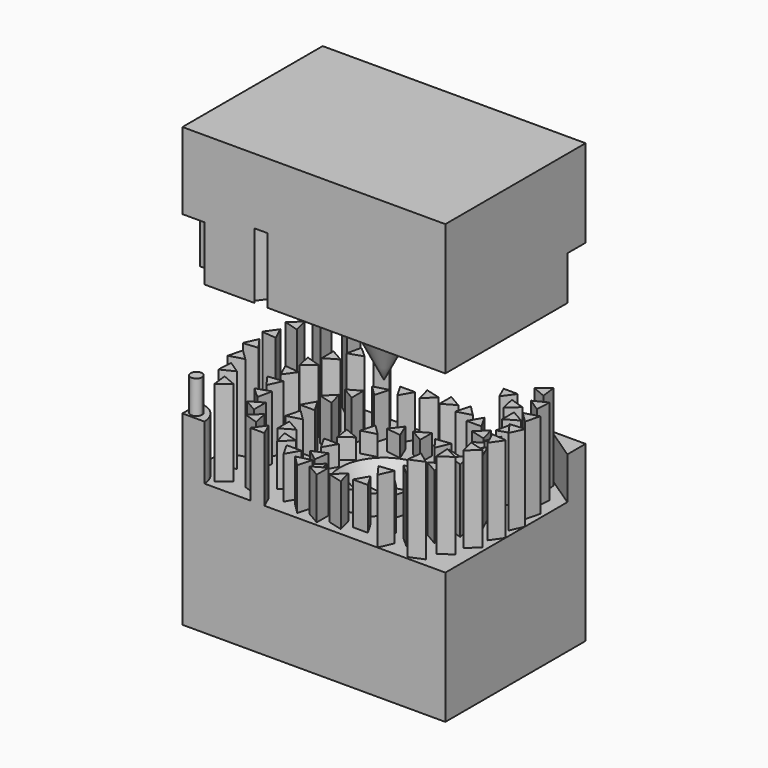
from build123d import *

# Parameters (mm, degrees)
F0_W      = 76.2
F0_H      = 50.8
F1_DEPTH  = 38.1
F3_W      = 76.2
F3_H      = 50.8
F4_DEPTH  = 38.1
F5_R      = 12.192
F13_DEPTH = 6.35
F16_DEPTH = 12.7
F17_DEPTH = 19.05
F18_DEPTH = 25.4
F20_DEPTH = 15.875
F21_DEPTH = 25.908
F23_DEPTH = 25.4
F24_DEPTH = 15.8242
F26_DEPTH = 12.7
F29_DEPTH = 5.842
F30_DEPTH = 12.192
F31_DEPTH = 18.542
F32_DEPTH = 24.892
F33_DEPTH = 12.192


# Not quite as in the source:
# - a feature names something its author has since deleted; it is built from what else it names


with BuildPart() as f1:
    # F0 (on Top) → F1 (new body)
    with BuildSketch(Plane.XY):
        Rectangle(F0_W, F0_H)
    extrude(amount=F1_DEPTH)

    # F14 (on 3pt) → F15 (revolve, cut)
    with BuildSketch(Plane(origin=(0, 0, 0), x_dir=(0, -1, 0), z_dir=(-1, 0, 0))):
        Polygon((0, 12.7), (0, 38.0711555481), (0, 38.1), (-12.7, 38.1), align=None)
    revolve(axis=Axis((0, 0, 25.4), (0, 0, -1)), mode=Mode.SUBTRACT)

    # F22 (on face) → F23 (join)
    with BuildSketch(Plane.XY.offset(38.1)):
        with BuildLine():
            Line((-37.0223692655, -24.3223692655), (-34.687502674, -21.987502674))
            ThreePointArc((-34.687502674, -21.987502674), (-37.0223692655, -21.987502674), (-37.0223692655, -24.3223692655))
        make_face()
        with BuildLine():
            ThreePointArc((-34.2039359697, -23.1549359697), (-34.3296108616, -22.5231256229), (-34.687502674, -21.987502674))
            Line((-34.687502674, -21.987502674), (-37.0223692655, -24.3223692655))
            ThreePointArc((-37.0223692655, -24.3223692655), (-35.2231256229, -24.6802610779), (-34.2039359697, -23.1549359697))
        make_face()
    extrude(amount=F23_DEPTH)

    # F22 (on face) → F24 (join)
    with BuildSketch(Plane.XY.offset(38.1)):
        with BuildLine():
            Line((-34.687502674, -21.987502674), (-33.6098719395, -20.9098719395))
            ThreePointArc((-33.6098719395, -20.9098719395), (-35.6699602045, -19.5333649686), (-38.1, -19.05))
            Line((-38.1, -19.05), (-38.1, -25.4))
            Line((-38.1, -25.4), (-37.0223692655, -24.3223692655))
            ThreePointArc((-37.0223692655, -24.3223692655), (-37.0223692655, -21.987502674), (-34.687502674, -21.987502674))
        make_face()
        with BuildLine():
            Line((-38.1, -25.4), (-31.75, -25.4))
            ThreePointArc((-31.75, -25.4), (-32.2333649686, -22.9699602045), (-33.6098719395, -20.9098719395))
            Line((-33.6098719395, -20.9098719395), (-34.687502674, -21.987502674))
            ThreePointArc((-34.687502674, -21.987502674), (-34.3296108616, -22.5231256229), (-34.2039359697, -23.1549359697))
            ThreePointArc((-34.2039359697, -23.1549359697), (-35.2231256229, -24.6802610779), (-37.0223692655, -24.3223692655))
            Line((-37.0223692655, -24.3223692655), (-38.1, -25.4))
        make_face()
    extrude(amount=F24_DEPTH)

    # F28 (on face) → F29 (join)
    with BuildSketch(Plane.XY.offset(38.1)):
        Polygon((-5.0058819788, 12.0852681648), (-6.6583090397, 16.0745799862), (-9.2869408902, 12.6488802628), align=None)
        Polygon((-9.2496638047, 9.2496638047), (-12.3029508859, 12.3029508859), (-13.4205315226, 8.1320831679), align=None)
        Polygon((5.0058819788, 12.0852681648), (6.6583090397, 16.0745799862), (2.3772501283, 15.5109678882), align=None)
        Polygon((9.2496638047, 9.2496638047), (12.3029508859, 12.3029508859), (8.1320831679, 13.4205315226), align=None)
        Polygon((12.0852681648, -5.0058819788), (16.0745799862, -6.6583090397), (15.5109678882, -2.3772501283), align=None)
        Polygon((12.0852681648, 5.0058819788), (16.0745799862, 6.6583090397), (12.6488802628, 9.2869408902), align=None)
        Polygon((13.081, 0), (17.399, 0), (15.24, 3.7394976935), align=None)
        Polygon((9.2496638047, -9.2496638047), (12.3029508859, -12.3029508859), (13.4205315226, -8.1320831679), align=None)
        Polygon((5.0058819788, -12.0852681648), (6.6583090397, -16.0745799862), (9.2869408902, -12.6488802628), align=None)
        Polygon((0, -13.081), (0, -17.399), (3.7394976935, -15.24), align=None)
        Polygon((-5.0058819788, -12.0852681648), (-6.6583090397, -16.0745799862), (-2.3772501283, -15.5109678882), align=None)
        Polygon((-9.2496638047, -9.2496638047), (-12.3029508859, -12.3029508859), (-8.1320831679, -13.4205315226), align=None)
        Polygon((-12.0852681648, -5.0058819788), (-16.0745799862, -6.6583090397), (-12.6488802628, -9.2869408902), align=None)
        Polygon((-13.081, 0), (-17.399, 0), (-15.24, -3.7394976935), align=None)
        Polygon((-12.0852681648, 5.0058819788), (-16.0745799862, 6.6583090397), (-15.5109678882, 2.3772501283), align=None)
        Polygon((-3.7394976935, 15.24), (0, 13.081), (0, 17.399), align=None)
    extrude(amount=F29_DEPTH)

    # F28 (on face) → F30 (join)
    with BuildSketch(Plane.XY.offset(38.1)):
        Polygon((-19.3822676303, 5.193462959), (-20.4998482671, 9.3643306769), (-23.5531353482, 6.3110435958), align=None)
        Polygon((-17.3776657523, 10.033), (-17.3776657523, 14.351), (-21.1171634459, 12.192), align=None)
        Polygon((-14.1888046713, 14.1888046713), (-13.0712240345, 18.3596723892), (-17.2420917525, 17.2420917525), align=None)
        Polygon((-20.066, 0), (-22.225, 3.7394976935), (-24.384, 0), align=None)
        Polygon((-19.3822676303, -5.193462959), (-22.4355547115, -2.1401758779), (-23.5531353482, -6.3110435958), align=None)
        Polygon((-17.3776657523, -10.033), (-21.1171634459, -7.874), (-21.1171634459, -12.192), align=None)
        Polygon((-14.1888046713, -14.1888046713), (-18.3596723892, -13.0712240345), (-17.2420917525, -17.2420917525), align=None)
        Polygon((-10.033, -17.3776657523), (-14.351, -17.3776657523), (-12.192, -21.1171634459), align=None)
        Polygon((-5.193462959, -19.3822676303), (-9.3643306769, -20.4998482671), (-6.3110435958, -23.5531353482), align=None)
        Polygon((-10.033, 17.3776657523), (-7.874, 21.1171634459), (-12.192, 21.1171634459), align=None)
        Polygon((-5.193462959, 19.3822676303), (-2.1401758779, 22.4355547115), (-6.3110435958, 23.5531353482), align=None)
        Polygon((0, 24.384), (0, 20.066), (3.7394976935, 22.225), align=None)
        Polygon((5.193462959, 19.3822676303), (9.3643306769, 20.4998482671), (6.3110435958, 23.5531353482), align=None)
        Polygon((10.033, 17.3776657523), (14.351, 17.3776657523), (12.192, 21.1171634459), align=None)
        Polygon((14.1888046713, 14.1888046713), (18.3596723892, 13.0712240345), (17.2420917525, 17.2420917525), align=None)
        Polygon((17.3776657523, 10.033), (21.1171634459, 7.874), (21.1171634459, 12.192), align=None)
        Polygon((19.3822676303, 5.193462959), (22.4355547115, 2.1401758779), (23.5531353482, 6.3110435958), align=None)
        Polygon((20.066, 0), (22.225, -3.7394976935), (24.384, 0), align=None)
        Polygon((19.3822676303, -5.193462959), (20.4998482671, -9.3643306769), (23.5531353482, -6.3110435958), align=None)
        Polygon((17.3776657523, -10.033), (17.3776657523, -14.351), (21.1171634459, -12.192), align=None)
        Polygon((14.1888046713, -14.1888046713), (13.0712240345, -18.3596723892), (17.2420917525, -17.2420917525), align=None)
        Polygon((10.033, -17.3776657523), (7.874, -21.1171634459), (12.192, -21.1171634459), align=None)
        Polygon((5.193462959, -19.3822676303), (2.1401758779, -22.4355547115), (6.3110435958, -23.5531353482), align=None)
        Polygon((0, -20.066), (-3.7394976935, -22.225), (0, -24.384), align=None)
    extrude(amount=F30_DEPTH)

    # F28 (on face) → F31 (join)
    with BuildSketch(Plane.XY.offset(38.1)):
        Polygon((18.2294342554, 25.4), (14.3350747947, 25.4), (15.9001788598, 21.8847187148), (18.4382355792, 25.3780540965), align=None)
        Polygon((19.205047993, 22.3242933726), (20.102810674, 18.1006520326), (23.3117100304, 20.9899579909), align=None)
        Polygon((23.4268531978, 17.8435), (23.4268531978, 13.5255), (27.1663508913, 15.6845), align=None)
        Polygon((26.6247925033, 12.5828600548), (25.7270298223, 8.3592187148), (29.8336918597, 9.6935540965), align=None)
        Polygon((28.6591006164, 6.772288746), (26.9028117916, 2.8275994599), (31.1971573358, 3.2789533642), align=None)
        Polygon((29.440868511, 0.6657359219), (26.9028117916, -2.8275994599), (31.1971573358, -3.2789533642), align=None)
        Polygon((28.9359291787, -5.4699127566), (25.7270298223, -8.3592187148), (29.8336918597, -9.6935540965), align=None)
        Polygon((27.1663508913, -11.3665), (23.4268531978, -13.5255), (27.1663508913, -15.6845), align=None)
        Polygon((24.2094727114, -16.7663166509), (20.102810674, -18.1006520326), (23.3117100304, -20.9899579909), align=None)
        Polygon((20.194524404, -21.4333648104), (15.9001788598, -21.8847187148), (18.4382355792, -25.3780540965), align=None)
        Polygon((-18.4382355792, -25.3780540965), (-18.2294342554, -25.4), (-14.3350747947, -25.4), (-15.9001788598, -21.8847187148), align=None)
        Polygon((-19.205047993, -22.3242933726), (-20.102810674, -18.1006520326), (-23.3117100304, -20.9899579909), align=None)
        Polygon((-23.4268531978, -17.8435), (-23.4268531978, -13.5255), (-27.1663508913, -15.6845), align=None)
        Polygon((-26.6247925033, -12.5828600548), (-25.7270298223, -8.3592187148), (-29.8336918597, -9.6935540965), align=None)
        Polygon((-28.6591006164, -6.772288746), (-26.9028117916, -2.8275994599), (-31.1971573358, -3.2789533642), align=None)
        Polygon((-29.440868511, -0.6657359219), (-26.9028117916, 2.8275994599), (-31.1971573358, 3.2789533642), align=None)
        Polygon((-28.9359291787, 5.4699127566), (-25.7270298223, 8.3592187148), (-29.8336918597, 9.6935540965), align=None)
        Polygon((-27.1663508913, 11.3665), (-23.4268531978, 13.5255), (-27.1663508913, 15.6845), align=None)
        Polygon((-24.2094727114, 16.7663166509), (-20.102810674, 18.1006520326), (-23.3117100304, 20.9899579909), align=None)
        Polygon((-20.194524404, 21.4333648104), (-15.9001788598, 21.8847187148), (-18.4382355792, 25.3780540965), align=None)
    extrude(amount=F31_DEPTH)

    # F28 (on face) → F32 (join)
    with BuildSketch(Plane.XY.offset(38.1)):
        Polygon((-27.1613143477, 20.5112724838), (-26.6306827086, 24.7965442446), (-30.6071527351, 23.1134488437), align=None)
        Polygon((-30.4677777846, 15.1711506772), (-30.7335977772, 19.4809608507), (-34.3330928766, 17.0958488975), align=None)
        Polygon((-32.736697591, 9.3143935301), (-33.7899170345, 13.5019766999), (-36.8898607183, 10.4960703212), align=None)
        Polygon((-35.6955611936, 7.0631989264), (-38.1, 3.666548848), (-38.1, 3.5304849218), (-33.8908084244, 3.1404458827), align=None)
        Polygon((-36.3856358284, 0.3838923849), (-38.1, -3.3423948867), (-38.1, -3.5304849218), (-33.8908084244, -3.1404458827), align=None)
        Polygon((-32.736697591, -9.3143935301), (-35.8366412748, -6.3084871514), (-36.8898607183, -10.4960703212), align=None)
        Polygon((-30.4677777846, -15.1711506772), (-34.0672728839, -12.786038724), (-34.3330928766, -17.0958488975), align=None)
        Polygon((-27.1613143477, -20.5112724838), (-31.1377843742, -18.8281770829), (-30.6071527351, -23.1134488437), align=None)
        Polygon((27.1613143477, -20.5112724838), (26.6306827086, -24.7965442446), (30.6071527351, -23.1134488437), align=None)
        Polygon((30.4677777846, -15.1711506772), (30.7335977772, -19.4809608507), (34.3330928766, -17.0958488975), align=None)
        Polygon((32.736697591, -9.3143935301), (33.7899170345, -13.5019766999), (36.8898607183, -10.4960703212), align=None)
        Polygon((38.1, -3.666548848), (38.1, -3.5304849218), (33.8908084244, -3.1404458827), (35.6955611936, -7.0631989264), align=None)
        Polygon((38.1, 3.3423948867), (38.1, 3.5304849218), (33.8908084244, 3.1404458827), (36.3856358284, -0.3838923849), align=None)
        Polygon((32.736697591, 9.3143935301), (35.8366412748, 6.3084871514), (36.8898607183, 10.4960703212), align=None)
        Polygon((30.4677777846, 15.1711506772), (34.0672728839, 12.786038724), (34.3330928766, 17.0958488975), align=None)
        Polygon((27.1613143477, 20.5112724838), (31.1377843742, 18.8281770829), (30.6071527351, 23.1134488437), align=None)
    extrude(amount=F32_DEPTH)

    # F27 (on face) → F33 (join)
    with BuildSketch(Plane.XY.offset(38.1)):
        Polygon((38.1, 25.4), (28.2770834, 25.4), (38.1, 18.796), align=None)
    extrude(amount=F33_DEPTH)


with BuildPart() as f4:
    # F3 (on offset) → F4 (new body)
    with BuildSketch(Plane.XY.offset(127)):
        Rectangle(F3_W, F3_H)
    extrude(amount=-F4_DEPTH)

    # F5 (on face) → F8 section 0
    with BuildSketch(Plane(origin=(0, 0, 88.9), x_dir=(1, 0, 0), z_dir=(0, 0, -1)), mode=Mode.PRIVATE) as f8_s0:
        Circle(F5_R)
    loft([f8_s0.sketch, Vertex(0, 0, 64.516)])

    # F12 (on face) → F13 (cut)
    with BuildSketch(Plane(origin=(0, 0, 88.9), x_dir=(1, 0, 0), z_dir=(0, 0, -1))):
        Polygon((0, 17.272), (0, 12.192), (4.3994090512, 14.732), align=None)
        Polygon((-6.6097082438, 15.9572472855), (-4.6656764074, 11.2639392604), (-1.573168348, 15.2941742291), align=None)
        Polygon((-12.2131483247, 12.2131483247), (-8.6210458762, 8.6210458762), (-7.3062451271, 13.5279490738), align=None)
        Polygon((-15.9572472855, 6.6097082438), (-11.2639392604, 4.6656764074), (-11.9270123169, 9.7022163032), align=None)
        Polygon((-17.272, 0), (-12.192, 0), (-14.732, 4.3994090512), align=None)
        Polygon((-15.9572472855, -6.6097082438), (-11.2639392604, -4.6656764074), (-15.2941742291, -1.573168348), align=None)
        Polygon((-12.2131483247, -12.2131483247), (-8.6210458762, -8.6210458762), (-13.5279490738, -7.3062451271), align=None)
        Polygon((-6.6097082438, -15.9572472855), (-4.6656764074, -11.2639392604), (-9.7022163032, -11.9270123169), align=None)
        Polygon((0, -17.272), (0, -12.192), (-4.3994090512, -14.732), align=None)
        Polygon((6.6097082438, -15.9572472855), (4.6656764074, -11.2639392604), (1.573168348, -15.2941742291), align=None)
        Polygon((12.2131483247, -12.2131483247), (8.6210458762, -8.6210458762), (7.3062451271, -13.5279490738), align=None)
        Polygon((15.9572472855, -6.6097082438), (11.2639392604, -4.6656764074), (11.9270123169, -9.7022163032), align=None)
        Polygon((15.9572472855, 6.6097082438), (11.2639392604, 4.6656764074), (15.2941742291, 1.573168348), align=None)
        Polygon((17.272, 0), (12.192, 0), (14.732, -4.3994090512), align=None)
        Polygon((12.2131483247, 12.2131483247), (8.6210458762, 8.6210458762), (13.5279490738, 7.3062451271), align=None)
        Polygon((6.6097082438, 15.9572472855), (4.6656764074, 11.2639392604), (9.7022163032, 11.9270123169), align=None)
    extrude(amount=-F13_DEPTH, mode=Mode.SUBTRACT)

    # F12 (on face) → F16 (cut)
    with BuildSketch(Plane(origin=(0, 0, 88.9), x_dir=(1, 0, 0), z_dir=(0, 0, -1))):
        Polygon((-4.9633728279, 18.5235595707), (-6.2781735771, 23.4304627683), (-9.8702760255, 19.8383603199), align=None)
        Polygon((-9.5885, 16.6077691684), (-12.1285, 21.0071782196), (-14.6685, 16.6077691684), align=None)
        Polygon((-13.5601867428, 13.5601867428), (-17.1522891912, 17.1522891912), (-18.4670899404, 12.2453859937), align=None)
        Polygon((-16.6077691684, 9.5885), (-21.0071782196, 12.1285), (-21.0071782196, 7.0485), align=None)
        Polygon((-18.5235595707, 4.9633728279), (-23.4304627683, 6.2781735771), (-22.1156620192, 1.3712703795), align=None)
        Polygon((-19.177, 0), (-24.257, 0), (-21.717, -4.3994090512), align=None)
        Polygon((-18.5235595707, -4.9633728279), (-23.4304627683, -6.2781735771), (-19.8383603199, -9.8702760255), align=None)
        Polygon((-16.6077691684, -9.5885), (-21.0071782196, -12.1285), (-16.6077691684, -14.6685), align=None)
        Polygon((-13.5601867428, -13.5601867428), (-17.1522891912, -17.1522891912), (-12.2453859937, -18.4670899404), align=None)
        Polygon((-9.5885, -16.6077691684), (-12.1285, -21.0071782196), (-7.0485, -21.0071782196), align=None)
        Polygon((-4.9633728279, -18.5235595707), (-6.2781735771, -23.4304627683), (-1.3712703795, -22.1156620192), align=None)
        Polygon((0, -19.177), (0, -24.257), (4.3994090512, -21.717), align=None)
        Polygon((4.9633728279, -18.5235595707), (6.2781735771, -23.4304627683), (9.8702760255, -19.8383603199), align=None)
        Polygon((9.5885, -16.6077691684), (12.1285, -21.0071782196), (14.6685, -16.6077691684), align=None)
        Polygon((13.5601867428, -13.5601867428), (17.1522891912, -17.1522891912), (18.4670899404, -12.2453859937), align=None)
        Polygon((16.6077691684, -9.5885), (21.0071782196, -12.1285), (21.0071782196, -7.0485), align=None)
        Polygon((4.9633728279, 18.5235595707), (6.2781735771, 23.4304627683), (1.3712703795, 22.1156620192), align=None)
        Polygon((9.5885, 16.6077691684), (12.1285, 21.0071782196), (7.0485, 21.0071782196), align=None)
        Polygon((13.5601867428, 13.5601867428), (17.1522891912, 17.1522891912), (12.2453859937, 18.4670899404), align=None)
        Polygon((16.6077691684, 9.5885), (21.0071782196, 12.1285), (16.6077691684, 14.6685), align=None)
        Polygon((18.5235595707, 4.9633728279), (23.4304627683, 6.2781735771), (19.8383603199, 9.8702760255), align=None)
        Polygon((19.177, 0), (24.257, 0), (21.717, 4.3994090512), align=None)
        Polygon((18.5235595707, -4.9633728279), (23.4304627683, -6.2781735771), (22.1156620192, -1.3712703795), align=None)
        Polygon((-4.3994090512, 21.717), (0, 19.177), (0, 24.257), align=None)
    extrude(amount=-F16_DEPTH, mode=Mode.SUBTRACT)

    # F12 (on face) → F17 (cut)
    with BuildSketch(Plane(origin=(0, 0, 88.9), x_dir=(1, 0, 0), z_dir=(0, 0, -1))):
        Polygon((-15.3776377705, 21.1655026068), (-13.4923180632, 25.4), (-17.1772306466, 25.4), (-18.3635868521, 25.2753089383), align=None)
        Polygon((12.707266203, 28.5409871877), (11.3088086068, 25.4), (14.9893269747, 25.4), align=None)
        Polygon((13.4923180632, -25.4), (17.1772306466, -25.4), (18.3635868521, -25.2753089383), (15.3776377705, -21.1655026068), align=None)
        Polygon((-23.2173306376, 20.9049784039), (-19.4421549241, 17.5057949236), (-18.3859635348, 22.4747847353), align=None)
        Polygon((-27.056365665, 15.621), (-22.6569566138, 13.081), (-22.6569566138, 18.161), align=None)
        Polygon((-29.7129076821, 9.6543089383), (-24.8815405793, 8.0845026068), (-25.9377319687, 13.0534924186), align=None)
        Polygon((-31.0708530551, 3.2656782494), (-26.0186818266, 2.734673656), (-28.0849039734, 7.3754845808), align=None)
        Polygon((-31.0708530551, -3.2656782494), (-26.0186818266, -2.734673656), (-29.0046309083, 1.3751326754), align=None)
        Polygon((-29.7129076821, -9.6543089383), (-24.8815405793, -8.0845026068), (-28.6567162927, -4.6853191265), align=None)
        Polygon((-27.056365665, -15.621), (-22.6569566138, -13.081), (-27.056365665, -10.541), align=None)
        Polygon((-23.2173306376, -20.9049784039), (-19.4421549241, -17.5057949236), (-24.2735220269, -15.9359885921), align=None)
        Polygon((-18.3635868521, -25.2753089383), (-15.3776377705, -21.1655026068), (-20.4298089989, -20.6344980134), align=None)
        Polygon((-6.4955770445, -30.5592873421), (-5.4393856552, -25.5902975304), (-10.270752758, -27.1601038618), align=None)
        Polygon((23.2173306376, -20.9049784039), (19.4421549241, -17.5057949236), (18.3859635348, -22.4747847353), align=None)
        Polygon((27.056365665, -15.621), (22.6569566138, -13.081), (22.6569566138, -18.161), align=None)
        Polygon((29.7129076821, -9.6543089383), (24.8815405793, -8.0845026068), (25.9377319687, -13.0534924186), align=None)
        Polygon((31.0708530551, -3.2656782494), (26.0186818266, -2.734673656), (28.0849039734, -7.3754845808), align=None)
        Polygon((31.0708530551, 3.2656782494), (26.0186818266, 2.734673656), (29.0046309083, -1.3751326754), align=None)
        Polygon((29.7129076821, 9.6543089383), (24.8815405793, 8.0845026068), (28.6567162927, 4.6853191265), align=None)
        Polygon((27.056365665, 15.621), (22.6569566138, 13.081), (27.056365665, 10.541), align=None)
        Polygon((23.2173306376, 20.9049784039), (19.4421549241, 17.5057949236), (24.2735220269, 15.9359885921), align=None)
        Polygon((18.3635868521, 25.2753089383), (15.3776377705, 21.1655026068), (20.4298089989, 20.6344980134), align=None)
        Polygon((6.4955770445, 30.5592873421), (5.4393856552, 25.5902975304), (10.270752758, 27.1601038618), align=None)
    extrude(amount=-F17_DEPTH, mode=Mode.SUBTRACT)

    # F12 (on face) → F18 (cut)
    with BuildSketch(Plane(origin=(0, 0, 88.9), x_dir=(1, 0, 0), z_dir=(0, 0, -1))):
        Polygon((-35.9406918052, -1.0878610036), (-33.0056007417, 3.0584193111), (-38.0639303572, 3.5271425772), align=None)
        Polygon((-35.1288392937, -7.673422892), (-33.0056007417, -3.0584193111), (-38.0639303572, -3.5271425772), align=None)
        Polygon((-33.1207162924, -13.997675567), (-31.8816345942, -9.0711071319), (-36.7677088616, -10.4613151215), align=None)
        Polygon((-29.9847070217, -19.8452541889), (-29.6719776185, -14.7748892789), (-34.2194071386, -17.0392401263), align=None)
        Polygon((-25.8276045161, -25.0170264812), (-26.4518770327, -19.9755302921), (-30.5058045472, -23.0369142449), align=None)
        Polygon((31.1300770638, -17.9954180557), (26.4518770327, -19.9755302921), (30.5058045472, -23.0369142449), align=None)
        Polygon((33.9066777355, -11.9688752163), (29.6719776185, -14.7748892789), (34.2194071386, -17.0392401263), align=None)
        Polygon((35.5286271634, -5.5347466864), (31.8816345942, -9.0711071319), (36.7677088616, -10.4613151215), align=None)
        Polygon((35.9406918052, 1.0878610036), (33.0056007417, -3.0584193111), (38.0639303572, -3.5271425772), align=None)
        Polygon((35.1288392937, 7.673422892), (33.0056007417, 3.0584193111), (38.0639303572, 3.5271425772), align=None)
        Polygon((33.1207162924, 13.997675567), (31.8816345942, 9.0711071319), (36.7677088616, 10.4613151215), align=None)
        Polygon((29.9847070217, 19.8452541889), (29.6719776185, 14.7748892789), (34.2194071386, 17.0392401263), align=None)
        Polygon((25.8276045161, 25.0170264812), (26.4518770327, 19.9755302921), (30.5058045472, 23.0369142449), align=None)
        Polygon((-31.1300770638, 17.9954180557), (-26.4518770327, 19.9755302921), (-30.5058045472, 23.0369142449), align=None)
        Polygon((-33.9066777355, 11.9688752163), (-29.6719776185, 14.7748892789), (-34.2194071386, 17.0392401263), align=None)
        Polygon((-35.5286271634, 5.5347466864), (-31.8816345942, 9.0711071319), (-36.7677088616, 10.4613151215), align=None)
    extrude(amount=-F18_DEPTH, mode=Mode.SUBTRACT)

    # F19 (on face) → F20 (cut)
    with BuildSketch(Plane(origin=(0, 0, 88.9), x_dir=(1, 0, 0), z_dir=(0, 0, -1))):
        with BuildLine():
            Line((-38.1, 25.4), (-38.1, 19.05))
            ThreePointArc((-38.1, 19.05), (-35.6699602045, 19.5333649686), (-33.6098719395, 20.9098719395))
            Line((-33.6098719395, 20.9098719395), (-34.5078975516, 21.8078975516))
            ThreePointArc((-34.5078975516, 21.8078975516), (-37.2019743879, 21.8078975516), (-37.2019743879, 24.5019743879))
            Line((-37.2019743879, 24.5019743879), (-38.1, 25.4))
        make_face()
        with BuildLine():
            Line((-34.5078975516, 21.8078975516), (-33.6098719395, 20.9098719395))
            ThreePointArc((-33.6098719395, 20.9098719395), (-32.2333649686, 22.9699602045), (-31.75, 25.4))
            Line((-31.75, 25.4), (-38.1, 25.4))
            Line((-38.1, 25.4), (-37.2019743879, 24.5019743879))
            ThreePointArc((-37.2019743879, 24.5019743879), (-35.1259240311, 24.9149264792), (-33.9499359697, 23.1549359697))
            ThreePointArc((-33.9499359697, 23.1549359697), (-34.0949454603, 22.4259240311), (-34.5078975516, 21.8078975516))
        make_face()
    extrude(amount=-F20_DEPTH, mode=Mode.SUBTRACT)

    # F19 (on face) → F21 (cut)
    with BuildSketch(Plane(origin=(0, 0, 88.9), x_dir=(1, 0, 0), z_dir=(0, 0, -1))):
        with BuildLine():
            ThreePointArc((-37.2019743879, 24.5019743879), (-37.2019743879, 21.8078975516), (-34.5078975516, 21.8078975516))
            Line((-34.5078975516, 21.8078975516), (-37.2019743879, 24.5019743879))
        make_face()
        with BuildLine():
            Line((-37.2019743879, 24.5019743879), (-34.5078975516, 21.8078975516))
            ThreePointArc((-34.5078975516, 21.8078975516), (-34.0949454603, 22.4259240311), (-33.9499359697, 23.1549359697))
            ThreePointArc((-33.9499359697, 23.1549359697), (-35.1259240311, 24.9149264792), (-37.2019743879, 24.5019743879))
        make_face()
    extrude(amount=-F21_DEPTH, mode=Mode.SUBTRACT)

    # F25 (on face) → F26 (cut)
    with BuildSketch(Plane(origin=(0, 0, 88.9), x_dir=(1, 0, 0), z_dir=(0, 0, -1))):
        Polygon((38.1, -25.4), (38.1, -18.796), (28.2770901057, -25.4), align=None)
    extrude(amount=-F26_DEPTH, mode=Mode.SUBTRACT)


solid = Compound([f1.part, f4.part])
